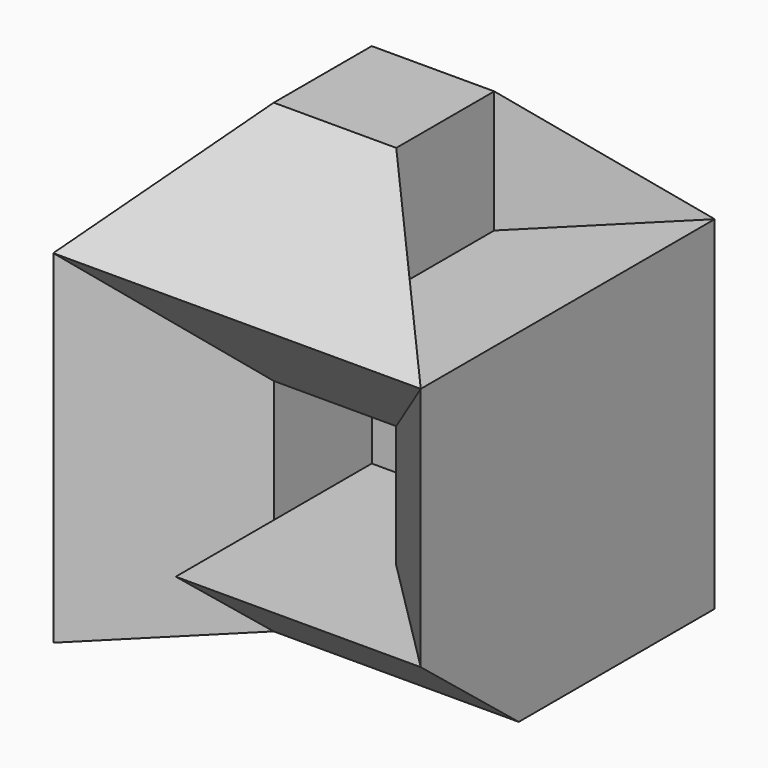
from build123d import *

# Parameters (mm, degrees)
F5_W           = 75
F5_H           = 75
F4_W           = 25
F4_H           = 25
F7_W           = 25
F7_H           = 25
F10_DEPTH      = 70.0000001
F11_DEPTH      = 70.00000015
F12_DEPTH      = 70.00000015
F14_DEPTH      = 37.5
F14_DEPTH_BACK = 12.5
F16_REACH      = 107.0166212872
F18_DEPTH      = 25


with BuildPart() as f6:
    # F5 (on offset) → F6 section 0
    with BuildSketch(Plane.XY.offset(70)):
        Rectangle(F5_W, F5_H)
    # F4 (on offset) → F6 section 1
    with BuildSketch(Plane.XY.offset(95)):
        Rectangle(F4_W, F4_H)
    loft()

    # F5 (on offset) → F8 section 0
    with BuildSketch(Plane.XY.offset(70)):
        Rectangle(F5_W, F5_H)
    # F7 (on offset) → F8 section 1
    with BuildSketch(Plane.XY.offset(45)):
        Rectangle(F7_W, F7_H)
    loft()

    # F9 (on Top) → F10 (join, through all)
    with BuildSketch(Plane.XY):
        Polygon((37.5, 37.5), (-37.5, 37.5), (-12.5, 12.5), (12.5, 12.5), align=None)
    extrude(amount=F10_DEPTH)

    # F9 (on Top) → F11 (join, through all)
    with BuildSketch(Plane.XY):
        Polygon((-37.5, 37.5), (-37.5, -37.5), (-12.5, -12.5), (-12.5, 12.5), align=None)
    extrude(amount=F11_DEPTH)

    # F9 (on Top) → F12 (join, through all)
    with BuildSketch(Plane.XY):
        Polygon((12.5, -12.5), (37.5, -37.5), (37.5, 37.5), (12.5, 12.5), align=None)
    extrude(amount=F12_DEPTH)

    # F13 (on Right) → F14 (join, two sides)
    with BuildSketch(Plane.YZ) as f14_sk:
        Polygon((-37.5, 20), (-12.5, 0), (12.5, 0), (12.5, 20), align=None)
    extrude(amount=F14_DEPTH)
    extrude(f14_sk.sketch, amount=-F14_DEPTH_BACK)

    f16_end = f6.faces().sort_by_distance((-25.9057971014, -25.9057971014, 29.2028985507))[0]
    # F15 (on face) → F16 (cut, up to a face of the model that its end follows)
    with BuildSketch(Plane.YZ.offset(37.5)):
        Polygon((-37.5, 0), (-12.5, 0), (-37.5, 20), align=None)
    f16_long = extrude(amount=-F16_REACH, mode=Mode.PRIVATE)
    add(split(f16_long, bisect_by=f16_end, keep=Keep.TOP, mode=Mode.PRIVATE), mode=Mode.SUBTRACT)

    # F17 (on offset) → F18 (cut, through all)
    with BuildSketch(Plane.XY.offset(95)):
        Polygon((12.5, 12.5), (12.5, -12.5), (37.5, -37.5), (37.5, -12.5), (37.5, 37.5), align=None)
    extrude(amount=-F18_DEPTH, mode=Mode.SUBTRACT)


solid = f6.part
